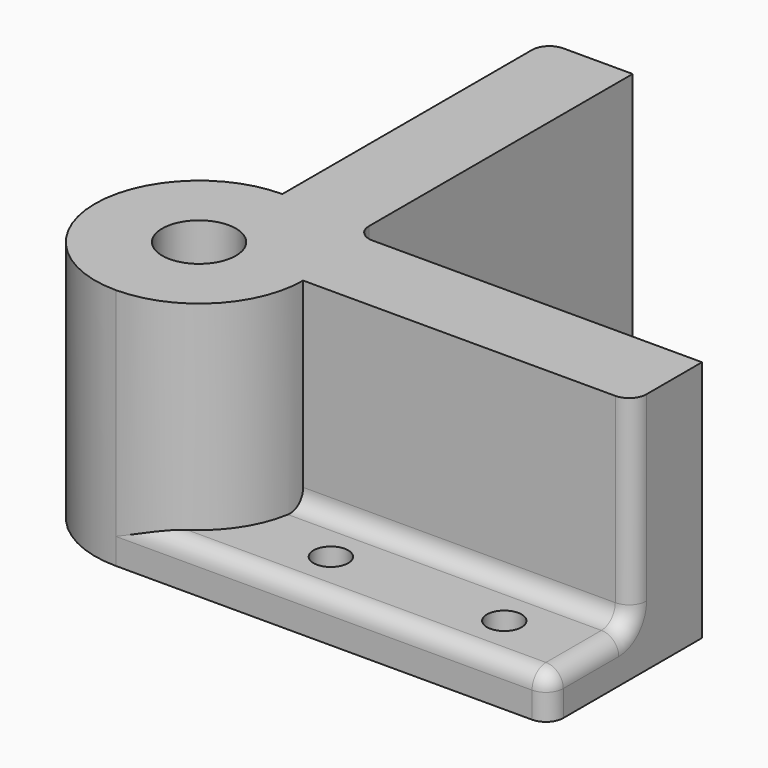
from build123d import *

# Parameters (mm, degrees)
F1_DEPTH     = 28
F0_R         = 2
F2_DEPTH     = 5
F3_DEPTH     = 5
F0_R_2       = 4.25
F4_DEPTH     = 28
F5_DEPTH     = 7
F6_T1_DEPTH  = 28
F6_T6_DEPTH  = 43
F6_S7_R      = 12
F6_T8_DEPTH  = 23
F6_T12_DEPTH = 43
F6_S13_R     = 12
F6_T14_DEPTH = 23
F6_T15_DEPTH = 5
F6_T20_DEPTH = 58.5
F6_S21_R     = 12
F6_T22_DEPTH = 31
F6_T26_DEPTH = 58.5
F6_S27_R     = 12
F6_T28_DEPTH = 31
F6_T33_DEPTH = 10
F6_T37_DEPTH = 63.5
F6_T44_DEPTH = 10
F6_T48_DEPTH = 63.5
F6_T51_DEPTH = 21
F6_T53_DEPTH = 8
F6_T55_DEPTH = 8
F6_S59_W     = 2.04
F6_S59_H     = 2.04
F6_T60_DEPTH = 2.04
F6_S65_W     = 2.04
F6_S65_H     = 2.04
F6_T66_DEPTH = 2.04
F6_T70_ANGLE = 90
F6_T72_ANGLE = 90


# Not quite as in the source:
# - a fillet or chamfer that OpenCascade refuses, or shapes differently, is made with other operations: its cross-section is extruded or revolved along the edge and cut away or added


with BuildPart() as f1:
    # F0 (on Top) → F1 (new body)
    with BuildSketch(Plane.XY):
        with BuildLine():
            Line((36.9490647506, 0), (-3.0509352494, 0))
            Line((-3.0509352494, 0), (-3.0509352494, 40))
            Line((-3.0509352494, 40), (-13.0509352494, 40))
            Line((-13.0509352494, 40), (-13.0509352494, 2))
            ThreePointArc((-13.0509352494, 2), (-21.5362166237, -1.5147186258), (-25.0509352494, -10))
            ThreePointArc((-25.0509352494, -10), (-21.5362166237, -18.4852813742), (-13.0509352494, -22))
            ThreePointArc((-13.0509352494, -22), (-4.5656538752, -18.4852813742), (-1.0509352494, -10))
            Line((-1.0509352494, -10), (36.9490647506, -10))
            Line((36.9490647506, -10), (36.9490647506, 0))
        make_face()
        Polygon((-5.7934883103, -8.1080528744), (-7.7837375065, -15.3391598531), (-15.0411844456, -17.2311069787), (-20.3083821886, -11.8919471256), (-18.3181329923, -4.6608401469), (-11.0606860532, -2.7688930213), align=None, mode=Mode.SUBTRACT)
    extrude(amount=F1_DEPTH)

    # F0 (on Top) → F2 (join)
    with BuildSketch(Plane.XY):
        with BuildLine():
            Line((-13.0509352494, 2), (-13.0509352494, 40))
            Line((-13.0509352494, 40), (-25.0509352494, 40))
            Line((-25.0509352494, 40), (-25.0509352494, -10))
            ThreePointArc((-25.0509352494, -10), (-21.5362166237, -1.5147186258), (-13.0509352494, 2))
        make_face()
        with Locations((-19.0509352494, 10)):
            Circle(F0_R, mode=Mode.SUBTRACT)
        with Locations((-19.0509352494, 30)):
            Circle(F0_R, mode=Mode.SUBTRACT)
    extrude(amount=F2_DEPTH)

    # F0 (on Top) → F3 (join)
    with BuildSketch(Plane.XY):
        with BuildLine():
            Line((36.9490647506, -22), (36.9490647506, -10))
            Line((36.9490647506, -10), (-1.0509352494, -10))
            ThreePointArc((-1.0509352494, -10), (-4.5656538752, -18.4852813742), (-13.0509352494, -22))
            Line((-13.0509352494, -22), (36.9490647506, -22))
        make_face()
        with Locations((6.9490647506, -16)):
            Circle(F0_R, mode=Mode.SUBTRACT)
        with Locations((26.9490647506, -16)):
            Circle(F0_R, mode=Mode.SUBTRACT)
    extrude(amount=F3_DEPTH)

    # F0 (on Top) → F4 (join)
    with BuildSketch(Plane.XY):
        Polygon((-15.0411844456, -17.2311069787), (-7.7837375065, -15.3391598531), (-5.7934883103, -8.1080528744), (-11.0606860532, -2.7688930213), (-18.3181329923, -4.6608401469), (-20.3083821886, -11.8919471256), align=None)
        with Locations((-13.0509352494, -10)):
            Circle(F0_R_2, mode=Mode.SUBTRACT)
    extrude(amount=F4_DEPTH)

    # F0 (on Top) → F5 (cut)
    with BuildSketch(Plane.XY):
        Polygon((-15.0411844456, -17.2311069787), (-7.7837375065, -15.3391598531), (-5.7934883103, -8.1080528744), (-11.0606860532, -2.7688930213), (-18.3181329923, -4.6608401469), (-20.3083821886, -11.8919471256), align=None)
        with Locations((-13.0509352494, -10)):
            Circle(F0_R_2, mode=Mode.SUBTRACT)
    extrude(amount=F5_DEPTH, mode=Mode.SUBTRACT)

    # F6: fillet of radius 2 on 11 edges, made by hand

    # F6_s2 → F6_t1 (join)
    with BuildSketch(Plane.XY):
        with BuildLine():
            ThreePointArc((-1.0509352494, 0), (-2.4651488118, 0.5857864376), (-3.0509352494, 2))
            Line((-3.0509352494, 2), (-3.0909352494, 2))
            Line((-3.0909352494, 2), (-3.0909352494, -0.04))
            Line((-3.0909352494, -0.04), (-1.0509352494, -0.04))
            Line((-1.0509352494, -0.04), (-1.0509352494, 0))
        make_face()
    extrude(amount=F6_T1_DEPTH)


with BuildPart() as f6_tool4:
    # F6_s5 → F6_t6 (new body)
    with BuildSketch(Plane.YZ.offset(36.9490647506)):
        with BuildLine():
            ThreePointArc((-10, 7), (-10.5857864376, 5.5857864376), (-12, 5))
            Line((-12, 5), (-12, 4.96))
            Line((-12, 4.96), (-9.96, 4.96))
            Line((-9.96, 4.96), (-9.96, 7))
            Line((-9.96, 7), (-10, 7))
        make_face()
    extrude(amount=-F6_T6_DEPTH)

    # F6_s7 → F6_t8 (cut, symmetric)
    with BuildSketch(Plane.XY.offset(6)):
        with Locations((-13.0509352494, -10)):
            Circle(F6_S7_R)
    extrude(amount=F6_T8_DEPTH, both=True, mode=Mode.SUBTRACT)


with BuildPart() as f1_1:
    add(f1.part)

    # F6_t3: union F6_tool4
    add(f6_tool4.part)


with BuildPart() as f6_tool10:
    # F6_s11 → F6_t12 (new body)
    with BuildSketch(Plane.XZ.offset(3)):
        with BuildLine():
            ThreePointArc((-13.0509352494, 7), (-13.6367216871, 5.5857864376), (-15.0509352494, 5))
            Line((-15.0509352494, 5), (-15.0509352494, 4.96))
            Line((-15.0509352494, 4.96), (-13.0109352494, 4.96))
            Line((-13.0109352494, 4.96), (-13.0109352494, 7))
            Line((-13.0109352494, 7), (-13.0509352494, 7))
        make_face()
    extrude(amount=-F6_T12_DEPTH)

    # F6_s13 → F6_t14 (cut, symmetric)
    with BuildSketch(Plane.XY.offset(6)):
        with Locations((-13.0509352494, -10)):
            Circle(F6_S13_R)
    extrude(amount=F6_T14_DEPTH, both=True, mode=Mode.SUBTRACT)


with BuildPart() as f1_2:
    add(f1_1.part)

    # F6_t9: union F6_tool10
    add(f6_tool10.part)

    # F6_s16 → F6_t15 (cut)
    with BuildSketch(Plane.XY):
        with BuildLine():
            ThreePointArc((36.9490647506, -20), (36.3632783129, -21.4142135624), (34.9490647506, -22))
            Line((34.9490647506, -22), (34.9490647506, -22.04))
            Line((34.9490647506, -22.04), (36.9890647506, -22.04))
            Line((36.9890647506, -22.04), (36.9890647506, -20))
            Line((36.9890647506, -20), (36.9490647506, -20))
        make_face()
        with BuildLine():
            ThreePointArc((-25.0509352494, 38), (-24.4651488118, 39.4142135624), (-23.0509352494, 40))
            Line((-23.0509352494, 40), (-23.0509352494, 40.04))
            Line((-23.0509352494, 40.04), (-25.0909352494, 40.04))
            Line((-25.0909352494, 40.04), (-25.0909352494, 38))
            Line((-25.0909352494, 38), (-25.0509352494, 38))
        make_face()
    extrude(amount=F6_T15_DEPTH, mode=Mode.SUBTRACT)


with BuildPart() as f6_tool18:
    # F6_s19 → F6_t20 (new body)
    with BuildSketch(Plane.YZ.offset(-21.5509352494)):
        with BuildLine():
            ThreePointArc((-22, 3), (-21.4142135624, 4.4142135624), (-20, 5))
            Line((-20, 5), (-20, 5.04))
            Line((-20, 5.04), (-22.04, 5.04))
            Line((-22.04, 5.04), (-22.04, 3))
            Line((-22.04, 3), (-22, 3))
        make_face()
    extrude(amount=F6_T20_DEPTH)

    # F6_s21 → F6_t22 (cut, symmetric)
    with BuildSketch(Plane.XY.offset(4)):
        with Locations((-13.0509352494, -10)):
            Circle(F6_S21_R)
    extrude(amount=F6_T22_DEPTH, both=True, mode=Mode.SUBTRACT)


with BuildPart() as f1_3:
    add(f1_2.part)

    # F6_t17: cut F6_tool18
    add(f6_tool18.part, mode=Mode.SUBTRACT)


with BuildPart() as f6_tool24:
    # F6_s25 → F6_t26 (new body)
    with BuildSketch(Plane.XZ.offset(-40)):
        with BuildLine():
            ThreePointArc((-25.0509352494, 3), (-24.4651488118, 4.4142135624), (-23.0509352494, 5))
            Line((-23.0509352494, 5), (-23.0509352494, 5.04))
            Line((-23.0509352494, 5.04), (-25.0909352494, 5.04))
            Line((-25.0909352494, 5.04), (-25.0909352494, 3))
            Line((-25.0909352494, 3), (-25.0509352494, 3))
        make_face()
    extrude(amount=F6_T26_DEPTH)

    # F6_s27 → F6_t28 (cut, symmetric)
    with BuildSketch(Plane.XY.offset(4)):
        with Locations((-13.0509352494, -10)):
            Circle(F6_S27_R)
    extrude(amount=F6_T28_DEPTH, both=True, mode=Mode.SUBTRACT)


with BuildPart() as f1_4:
    add(f1_3.part)

    # F6_t23: cut F6_tool24
    add(f6_tool24.part, mode=Mode.SUBTRACT)


with BuildPart() as f6_tool31:
    # F6_s32 → F6_t33 (new body)
    with BuildSketch(Plane.XY):
        with BuildLine():
            ThreePointArc((36.9490647506, -20), (36.3632783129, -21.4142135624), (34.9490647506, -22))
            Line((34.9490647506, -22), (34.9490647506, -22.04))
            Line((34.9490647506, -22.04), (36.9890647506, -22.04))
            Line((36.9890647506, -22.04), (36.9890647506, -20))
            Line((36.9890647506, -20), (36.9490647506, -20))
        make_face()
    extrude(amount=F6_T33_DEPTH)

    split(bisect_by=Plane.XY.offset(5), keep=Keep.TOP)


with BuildPart() as f6_tool35:
    # F6_s36 → F6_t37 (new body)
    with BuildSketch(Plane.YZ.offset(-21.5509352494)):
        with BuildLine():
            ThreePointArc((-22, 3), (-21.4142135624, 4.4142135624), (-20, 5))
            Line((-20, 5), (-20, 5.04))
            Line((-20, 5.04), (-22.04, 5.04))
            Line((-22.04, 5.04), (-22.04, 3))
            Line((-22.04, 3), (-22, 3))
        make_face()
    extrude(amount=F6_T37_DEPTH)

    split(bisect_by=Plane.YZ.offset(36.9490647506), keep=Keep.TOP)


with BuildPart() as f6_tool31_1:
    add(f6_tool31.part)

    # F6_t39: intersect F6_tool35
    add(f6_tool35.part, mode=Mode.INTERSECT)


with BuildPart() as f1_5:
    add(f1_4.part)

    # F6_t29: cut F6_tool31
    add(f6_tool31_1.part, mode=Mode.SUBTRACT)


with BuildPart() as f6_tool42:
    # F6_s43 → F6_t44 (new body)
    with BuildSketch(Plane.XY):
        with BuildLine():
            ThreePointArc((-25.0509352494, 38), (-24.4651488118, 39.4142135624), (-23.0509352494, 40))
            Line((-23.0509352494, 40), (-23.0509352494, 40.04))
            Line((-23.0509352494, 40.04), (-25.0909352494, 40.04))
            Line((-25.0909352494, 40.04), (-25.0909352494, 38))
            Line((-25.0909352494, 38), (-25.0509352494, 38))
        make_face()
    extrude(amount=F6_T44_DEPTH)

    split(bisect_by=Plane.XY.offset(5), keep=Keep.TOP)


with BuildPart() as f6_tool46:
    # F6_s47 → F6_t48 (new body)
    with BuildSketch(Plane.XZ.offset(-45)):
        with BuildLine():
            ThreePointArc((-25.0509352494, 3), (-24.4651488118, 4.4142135624), (-23.0509352494, 5))
            Line((-23.0509352494, 5), (-23.0509352494, 5.04))
            Line((-23.0509352494, 5.04), (-25.0909352494, 5.04))
            Line((-25.0909352494, 5.04), (-25.0909352494, 3))
            Line((-25.0909352494, 3), (-25.0509352494, 3))
        make_face()
    extrude(amount=F6_T48_DEPTH)

    split(bisect_by=Plane.XZ.offset(-40), keep=Keep.BOTTOM)


with BuildPart() as f6_tool42_1:
    add(f6_tool42.part)

    # F6_t50: intersect F6_tool46
    add(f6_tool46.part, mode=Mode.INTERSECT)


with BuildPart() as f1_6:
    add(f1_5.part)

    # F6_t40: cut F6_tool42
    add(f6_tool42_1.part, mode=Mode.SUBTRACT)

    # F6_s52 → F6_t51 (cut)
    with BuildSketch(Plane.XY.offset(7)):
        with BuildLine():
            ThreePointArc((36.9490647506, -8), (36.3632783129, -9.4142135624), (34.9490647506, -10))
            Line((34.9490647506, -10), (34.9490647506, -10.04))
            Line((34.9490647506, -10.04), (36.9890647506, -10.04))
            Line((36.9890647506, -10.04), (36.9890647506, -8))
            Line((36.9890647506, -8), (36.9490647506, -8))
        make_face()
        with BuildLine():
            ThreePointArc((-11.0509352494, 40), (-12.4651488118, 39.4142135624), (-13.0509352494, 38))
            Line((-13.0509352494, 38), (-13.0909352494, 38))
            Line((-13.0909352494, 38), (-13.0909352494, 40.04))
            Line((-13.0909352494, 40.04), (-11.0509352494, 40.04))
            Line((-11.0509352494, 40.04), (-11.0509352494, 40))
        make_face()
    extrude(amount=F6_T51_DEPTH, mode=Mode.SUBTRACT)

    # F6_s54 → F6_t53 (cut)
    with BuildSketch(Plane.XZ.offset(12)):
        with BuildLine():
            ThreePointArc((36.9490647506, 3), (36.3632783129, 4.4142135624), (34.9490647506, 5))
            Line((34.9490647506, 5), (34.9490647506, 5.04))
            Line((34.9490647506, 5.04), (36.9890647506, 5.04))
            Line((36.9890647506, 5.04), (36.9890647506, 3))
            Line((36.9890647506, 3), (36.9490647506, 3))
        make_face()
    extrude(amount=F6_T53_DEPTH, mode=Mode.SUBTRACT)

    # F6_s56 → F6_t55 (cut)
    with BuildSketch(Plane.YZ.offset(-23.0509352494)):
        with BuildLine():
            ThreePointArc((40, 3), (39.4142135624, 4.4142135624), (38, 5))
            Line((38, 5), (38, 5.04))
            Line((38, 5.04), (40.04, 5.04))
            Line((40.04, 5.04), (40.04, 3))
            Line((40.04, 3), (40, 3))
        make_face()
    extrude(amount=F6_T55_DEPTH, mode=Mode.SUBTRACT)


with BuildPart() as f6_tool58:
    # F6_s59 → F6_t60 (new body)
    with BuildSketch(Plane.XZ.offset(-38)):
        with Locations((-24.0709352494, 4.02)):
            Rectangle(F6_S59_W, F6_S59_H)
    extrude(amount=-F6_T60_DEPTH)

    # F6_s61 → F6_t62 (revolve, cut)
    with BuildSketch(Plane(origin=(-23.0509352494, 38, 3), x_dir=(0.7071067812, 0, -0.7071067812), z_dir=(0.7071067812, 0, 0.7071067812))):
        with BuildLine():
            ThreePointArc((0, -2), (2, 0), (0, 2))
            Line((0, 2), (0, -2))
        make_face()
    revolve(axis=Axis((-23.0509352494, 38, 3), (0, 1, 0)), mode=Mode.SUBTRACT)


with BuildPart() as f1_7:
    add(f1_6.part)

    # F6_t57: cut F6_tool58
    add(f6_tool58.part, mode=Mode.SUBTRACT)


with BuildPart() as f6_tool64:
    # F6_s65 → F6_t66 (new body)
    with BuildSketch(Plane.YZ.offset(34.9490647506)):
        with Locations((-21.02, 4.02)):
            Rectangle(F6_S65_W, F6_S65_H)
    extrude(amount=F6_T66_DEPTH)

    # F6_s67 → F6_t68 (revolve, cut)
    with BuildSketch(Plane(origin=(34.9490647506, -20, 3), x_dir=(0, 0.7071067812, -0.7071067812), z_dir=(0, -0.7071067812, -0.7071067812))):
        with BuildLine():
            ThreePointArc((0, -2), (2, 0), (0, 2))
            Line((0, 2), (0, -2))
        make_face()
    revolve(axis=Axis((34.9490647506, -20, 3), (1, 0, 0)), mode=Mode.SUBTRACT)


with BuildPart() as f1_8:
    add(f1_7.part)

    # F6_t63: cut F6_tool64
    add(f6_tool64.part, mode=Mode.SUBTRACT)

    # F6_s69 → F6_t70 (revolve, cut)
    with BuildSketch(Plane.XY.offset(7)):
        with BuildLine():
            ThreePointArc((-11.0509352494, 40), (-12.4651488118, 39.4142135624), (-13.0509352494, 38))
            Line((-13.0509352494, 38), (-13.0909352494, 38))
            Line((-13.0909352494, 38), (-13.0909352494, 40.04))
            Line((-13.0909352494, 40.04), (-11.0509352494, 40.04))
            Line((-11.0509352494, 40.04), (-11.0509352494, 40))
        make_face()
    revolve(axis=Axis((-15.0509352494, 40, 7), (0, 1, 0)), revolution_arc=F6_T70_ANGLE, mode=Mode.SUBTRACT)

    # F6_s71 → F6_t72 (revolve, cut)
    with BuildSketch(Plane.XY.offset(7)):
        with BuildLine():
            ThreePointArc((36.9490647506, -8), (36.3632783129, -9.4142135624), (34.9490647506, -10))
            Line((34.9490647506, -10), (34.9490647506, -10.04))
            Line((34.9490647506, -10.04), (36.9890647506, -10.04))
            Line((36.9890647506, -10.04), (36.9890647506, -8))
            Line((36.9890647506, -8), (36.9490647506, -8))
        make_face()
    revolve(axis=Axis((36.9490647506, -12, 7), (-1, 0, 0)), revolution_arc=F6_T72_ANGLE, mode=Mode.SUBTRACT)


solid = f1_8.part
